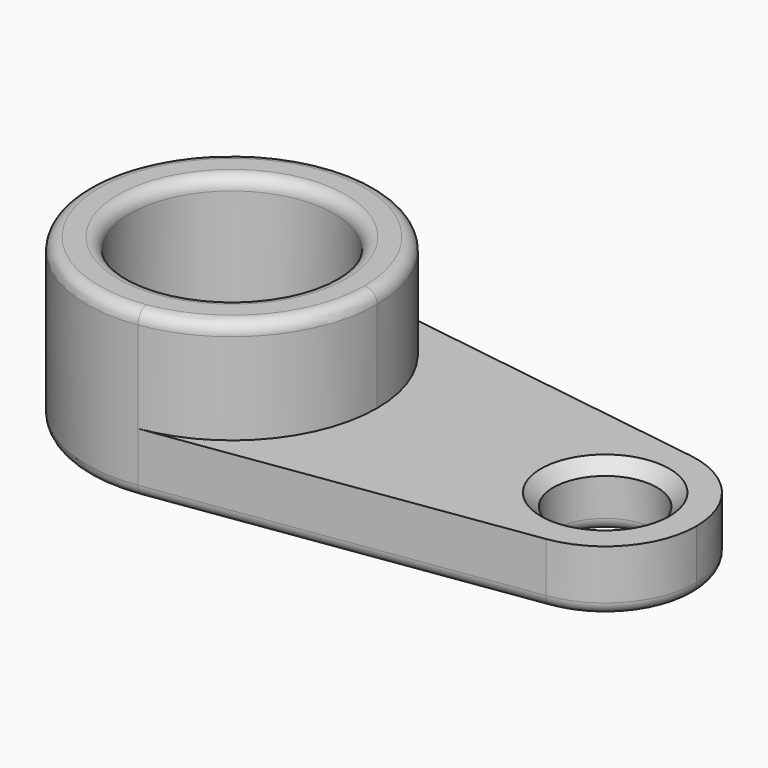
from build123d import *

# Parameters (mm, degrees)
F0_R     = 24.5
F0_R_2   = 12.5
F1_DEPTH = 15
F2_DEPTH = 25
F3_R     = 3
F4_SIZE  = 3


# Not quite as in the source:
# - a feature names something its author has since deleted; it is built from what else it names


with BuildPart() as f1:
    # F0 (on Top) → F1 (new body)
    with BuildSketch(Plane.XY):
        with BuildLine():
            ThreePointArc((35, 0), (26.4758800085, 22.8916530154), (5.0555555556, 34.6329519104))
            ThreePointArc((5.0555555556, 34.6329519104), (-35, 0), (5.0555555556, -34.6329519104))
            ThreePointArc((5.0555555556, -34.6329519104), (26.4758800085, -22.8916530154), (35, 0))
        make_face()
        Circle(F0_R, mode=Mode.SUBTRACT)
        with BuildLine():
            Line((93.1777777778, 21.7692840579), (5.0555555556, 34.6329519104))
            ThreePointArc((5.0555555556, 34.6329519104), (26.4758800085, 22.8916530154), (35, 0))
            ThreePointArc((35, 0), (26.4758800085, -22.8916530154), (5.0555555556, -34.6329519104))
            Line((5.0555555556, -34.6329519104), (93.1777777778, -21.7692840579))
            ThreePointArc((93.1777777778, -21.7692840579), (68, 0), (93.1777777778, 21.7692840579))
        make_face()
        with BuildLine():
            ThreePointArc((112, 0), (106.6419817196, 14.3890390383), (93.1777777778, 21.7692840579))
            ThreePointArc((93.1777777778, 21.7692840579), (68, 0), (93.1777777778, -21.7692840579))
            ThreePointArc((93.1777777778, -21.7692840579), (106.6419817196, -14.3890390383), (112, 0))
        make_face()
        with Locations((90, 0)):
            Circle(F0_R_2, mode=Mode.SUBTRACT)
    extrude(amount=-F1_DEPTH)

    # F0 (on Top) → F2 (join)
    with BuildSketch(Plane.XY):
        with BuildLine():
            ThreePointArc((35, 0), (26.4758800085, 22.8916530154), (5.0555555556, 34.6329519104))
            ThreePointArc((5.0555555556, 34.6329519104), (-35, 0), (5.0555555556, -34.6329519104))
            ThreePointArc((5.0555555556, -34.6329519104), (26.4758800085, -22.8916530154), (35, 0))
        make_face()
        Circle(F0_R, mode=Mode.SUBTRACT)
    extrude(amount=F2_DEPTH)

    # F3
    f3_edges = [f1.edges().sort_by_distance(p)[0] for p in [
        (-5.055556, 34.632952, 25),
        (-24.5, 0, 25),
        (-35, 0, -15),
        (49.116667, -28.201118, -15),
        (112, 0, -15),
        (49.116667, 28.201118, -15),
        (-24.5, 0, -15),
        (77.5, 0, -15),
    ]]
    fillet(f3_edges, radius=F3_R)

    # F4
    f4_edges = [f1.edges().sort_by_distance(p)[0] for p in [
        (77.5, 0, 0),
    ]]
    chamfer(f4_edges, length=F4_SIZE)


solid = f1.part
